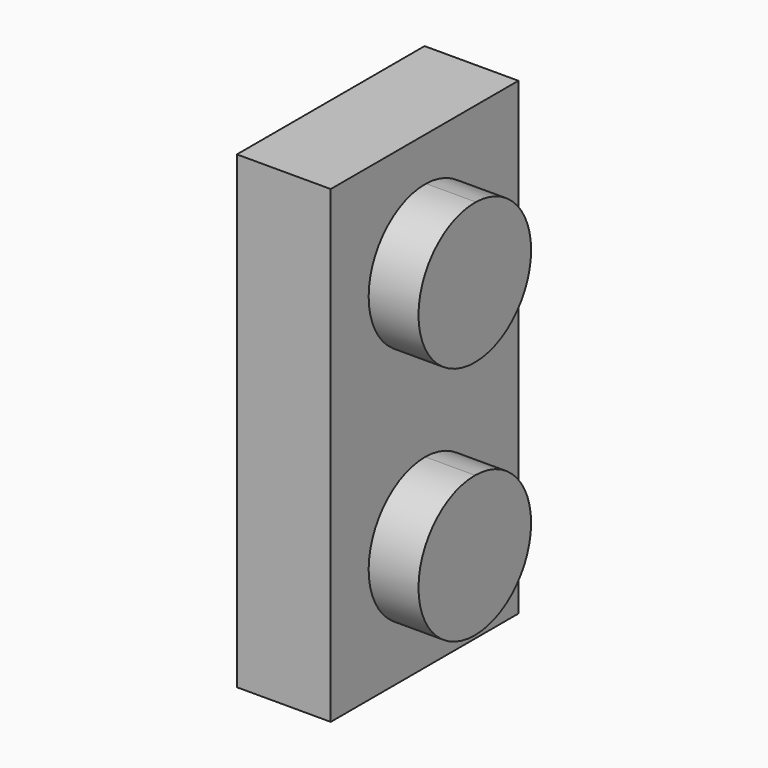
from build123d import *

# Parameters (mm, degrees)
F0_W     = 8
F0_H     = 16
F1_DEPTH = 3.2
F3_DEPTH = 1.7


# Not quite as in the source:
# - a feature names something its author has since deleted; it is built from what else it names


with BuildPart() as f1:
    # F0 (on Right) → F1 (new body)
    with BuildSketch(Plane.YZ):
        with Locations((4, 8)):
            Rectangle(F0_W, F0_H)
    extrude(amount=F1_DEPTH)

    # F2 (on face) → F3 (join)
    with BuildSketch(Plane.YZ.offset(3.2)):
        with BuildLine():
            ThreePointArc((4.0419005416, 9.7116244191), (5.7227796266, 10.4232962474), (6.4169111453, 12.1114943177))
            ThreePointArc((6.4169111453, 12.1114943177), (5.730047367, 13.7923168204), (4.0626075738, 14.5110592441))
            Line((4.0626075738, 14.5110592441), (4.0419005416, 9.7116244191))
        make_face()
        with BuildLine():
            Line((4.0419005416, 9.7116244191), (4.0626075738, 14.5110592441))
            ThreePointArc((4.0626075738, 14.5110592441), (1.6169334826, 12.1218489566), (4.0419005416, 9.7116244191))
        make_face()
        with BuildLine():
            ThreePointArc((6.4169111453, 3.9196317084), (5.7176243976, 5.6130231083), (4.0272657842, 6.3196093711))
            Line((4.0272657842, 6.3196093711), (4.0272298946, 6.3112909609))
            Line((4.0272298946, 6.3112909609), (4.0065565064, 1.5196540457))
            ThreePointArc((4.0065565064, 1.5196540457), (5.7103025452, 2.2189184561), (6.4169111453, 3.9196317084))
        make_face()
        with BuildLine():
            Line((4.0272298946, 6.3112909609), (4.0272657842, 6.3196093711))
            ThreePointArc((4.0272657842, 6.3196093711), (1.6169334826, 3.9299863473), (4.0065565064, 1.5196540457))
            Line((4.0065565064, 1.5196540457), (4.0272298946, 6.3112909609))
        make_face()
    extrude(amount=F3_DEPTH)


solid = f1.part
